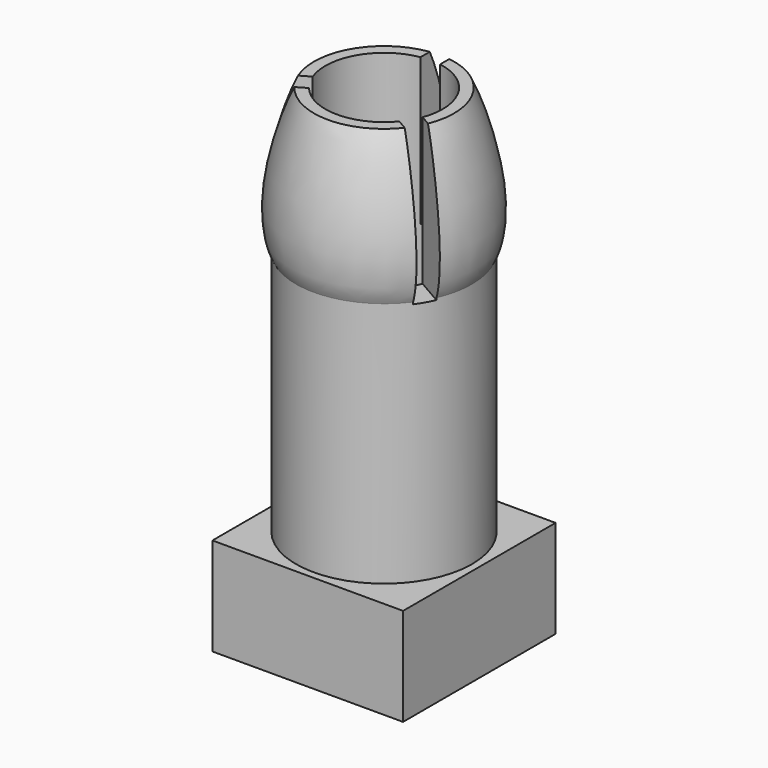
from build123d import *

# Parameters (mm, degrees)
F0_W         = 9.75
F0_H         = 9.75
F0_W_2       = 6
F0_H_2       = 6
F1_DEPTH     = 5
F4_W         = 1
F4_H         = 10.4783805975
F5_DEPTH     = 7.5
F6_T4_ANGLE  = 90
F6_T10_ANGLE = 90
F6_T16_ANGLE = 90
F6_T22_ANGLE = 90


# Not quite as in the source:
# - a fillet or chamfer that OpenCascade refuses, or shapes differently, is made with other operations: its cross-section is extruded or revolved along the edge and cut away or added


with BuildPart() as f1:
    # F0 (on Top) → F1 (new body)
    with BuildSketch(Plane.XY):
        Rectangle(F0_W, F0_H)
        Rectangle(F0_W_2, F0_H_2, mode=Mode.SUBTRACT)
    extrude(amount=F1_DEPTH)

    # F2 (on Front) → F3 (revolve)
    with BuildSketch(Plane.XZ):
        with BuildLine():
            Line((3, 25), (3, 5))
            Line((3, 5), (4.5, 5))
            Line((4.5, 5), (4.5, 17.5993331894))
            add(Edge.make_bspline(
                [(3.5845720258, 25), (4.1028451178, 23.9598143656), (5.5548848687, 19.7320627697), (4.5, 17.5993331894)],
                knots=[0, 0, 0, 0, 7.4570689696, 7.4570689696, 7.4570689696, 7.4570689696], degree=3))
            Line((3.5845720258, 25), (3, 25))
        make_face()
    revolve(axis=Axis((0, 0, 5.0040013157), (0, 0, -1)))

    # F4 (on face) → F5 (cut)
    with BuildSketch(Plane.XY.offset(25)):
        with Locations((0, 5.5278654333)):
            Rectangle(F4_W, F4_H)
        Polygon((0, -0.5773502692), (-0.5, 0.2886751346), (-9.574543788, -4.9505151642), (-9.074543788, -5.8165405679), align=None)
        Polygon((0.5, 0.2886751346), (-0.5, 0.2886751346), (0, -0.5773502692), align=None)
        Polygon((9.574543788, -4.9505151642), (0.5, 0.2886751346), (0, -0.5773502692), (9.074543788, -5.8165405679), align=None)
    extrude(amount=-F5_DEPTH, mode=Mode.SUBTRACT)

    # F6: chamfer of 1.24 on 1 edges, made by hand


with BuildPart() as f6_tool2:
    # F6_s3 → F6_t4 (revolve)
    with BuildSketch(Plane.YZ):
        Polygon((-3, 6.24), (-4.24, 5), (-3, 5), align=None)
    revolve(axis=Axis((0, 0, 5), (0, 0, -1)), revolution_arc=F6_T4_ANGLE)

    split(bisect_by=Plane.XZ.offset(3), keep=Keep.BOTTOM)

    split(bisect_by=Plane.YZ.offset(-3), keep=Keep.TOP)


with BuildPart() as f1_1:
    add(f1.part)

    # F6_t1: cut F6_tool2
    add(f6_tool2.part, mode=Mode.SUBTRACT)


with BuildPart() as f6_tool8:
    # F6_s9 → F6_t10 (revolve)
    with BuildSketch(Plane.XZ):
        Polygon((3, 6.24), (4.24, 5), (3, 5), align=None)
    revolve(axis=Axis((0, 0, 5), (0, 0, -1)), revolution_arc=F6_T10_ANGLE)

    split(bisect_by=Plane.YZ.offset(3), keep=Keep.BOTTOM)

    split(bisect_by=Plane.XZ.offset(3), keep=Keep.BOTTOM)


with BuildPart() as f1_2:
    add(f1_1.part)

    # F6_t7: cut F6_tool8
    add(f6_tool8.part, mode=Mode.SUBTRACT)


with BuildPart() as f6_tool14:
    # F6_s15 → F6_t16 (revolve)
    with BuildSketch(Plane.XZ):
        Polygon((-3, 6.24), (-4.24, 5), (-3, 5), align=None)
    revolve(axis=Axis((0, 0, 5), (0, 0, -1)), revolution_arc=F6_T16_ANGLE)

    split(bisect_by=Plane.YZ.offset(-3), keep=Keep.TOP)

    split(bisect_by=Plane.XZ.offset(-3), keep=Keep.TOP)


with BuildPart() as f1_3:
    add(f1_2.part)

    # F6_t13: cut F6_tool14
    add(f6_tool14.part, mode=Mode.SUBTRACT)


with BuildPart() as f6_tool20:
    # F6_s21 → F6_t22 (revolve)
    with BuildSketch(Plane.YZ):
        Polygon((3, 6.24), (4.24, 5), (3, 5), align=None)
    revolve(axis=Axis((0, 0, 5), (0, 0, -1)), revolution_arc=F6_T22_ANGLE)

    split(bisect_by=Plane.YZ.offset(3), keep=Keep.BOTTOM)

    split(bisect_by=Plane.XZ.offset(-3), keep=Keep.TOP)


with BuildPart() as f1_4:
    add(f1_3.part)

    # F6_t19: cut F6_tool20
    add(f6_tool20.part, mode=Mode.SUBTRACT)


solid = f1_4.part
